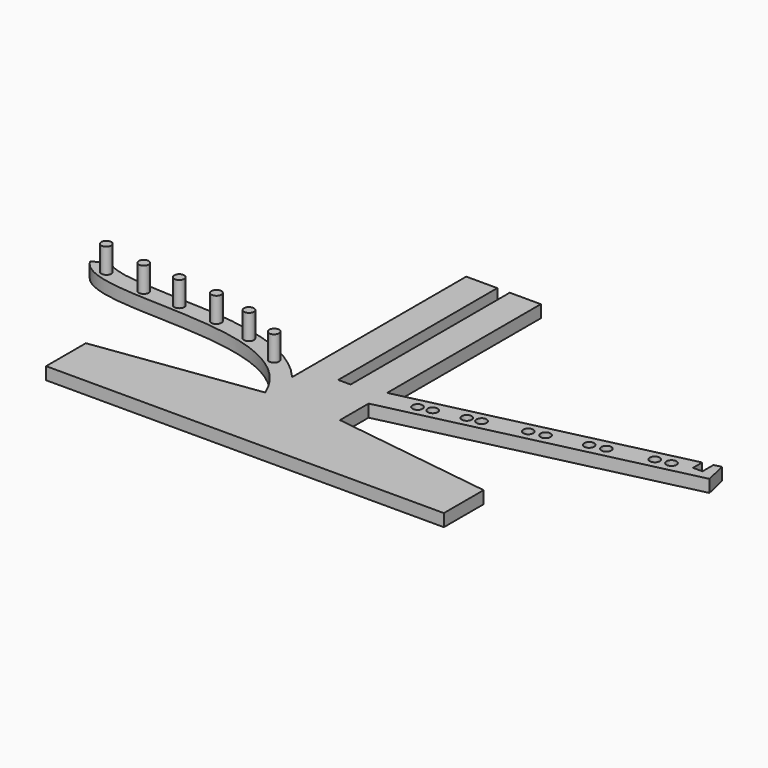
from build123d import *

# Parameters (mm, degrees)
F0_R     = 2
F1_DEPTH = 5
F2_D     = 4
F2_DEPTH = 10
F2_TIP   = 1.2017212381
F3_DEPTH = 15


# Not quite as in the source:
# - ends of sketch curves that miss each other by under 0.0002 mm in the source are joined
# - the dataset's text gives a spline's control points without its knots; the knots are read off the source's solid


with BuildPart() as f1:
    # F0 (on Top) → F1 (new body)
    with BuildSketch(Plane.XY):
        Polygon((-160, 0), (0, 0), (0, 20), (-65, 29), (-65, 43.4094795469), (-65, 52.718677739), (-65, 130), (-77.5, 130), (-77.5, 50), (-82.5, 50), (-82.5, 130), (-95, 130), (-95, 42.4402998717), (-95, 42.4395510141), (-95, 29), (-160, 20), align=None)
        with BuildLine():
            add(Edge.make_bspline(
                [(-95, 29), (-112.1026869317, 69.879398944), (-183.2138453119, 44.6590780371), (-193.7192612239, 64.3418715165)],
                knots=[0, 0, 0, 0, 104.8548540549, 104.8548540549, 104.8548540549, 104.8548540549], degree=3))
            Line((-95, 29), (-95, 42.4395510141))
            add(Edge.make_bspline(
                [(-95, 42.4395510141), (-96.2567038445, 43.9528858593), (-99.6573677898, 47.484596761), (-105.8513361132, 51.9891056969), (-113.4978559187, 55.6874902914), (-121.5446515491, 58.2622912897), (-129.8174188241, 59.9692128244), (-138.169171381, 61.0325579202), (-146.4541296432, 61.6510478997), (-154.5172718143, 62.00683513), (-162.1896252518, 62.271111182), (-169.2832883204, 62.6056387967), (-175.5824829207, 63.1564158073), (-179.9528366956, 63.8911416604), (-182.7618397147, 64.6491460265), (-184.483037472, 65.2820676907), (-185.7879555086, 65.9413674264), (-186.6785109442, 66.5698730777), (-187.2176454673, 67.115204059), (-187.4401377715, 67.4455917293), (-187.5371722477, 67.6255274527)],
                knots=[0.0840071742, 0.0840071742, 0.0840071742, 0.0840071742, 0.125, 0.1875, 0.25, 0.3125, 0.375, 0.4375, 0.5, 0.5625, 0.625, 0.6875, 0.75, 0.8125, 0.84375, 0.875, 0.90625, 0.9375, 0.96875, 0.9992998663, 0.9992998663, 0.9992998663, 0.9992998663], degree=3))
            Line((-187.5371722477, 67.6255274527), (-193.7192612239, 64.3418715165))
        make_face()
        with Locations((-185.2389183558, 61.8432959386)):
            Circle(F0_R, mode=Mode.SUBTRACT)
        with Locations((-167.974160698, 59.0616882791)):
            Circle(F0_R, mode=Mode.SUBTRACT)
        with Locations((-153.1901955605, 58.4377646446)):
            Circle(F0_R, mode=Mode.SUBTRACT)
        with Locations((-137.3645175282, 57.3560006478)):
            Circle(F0_R, mode=Mode.SUBTRACT)
        with Locations((-106.7991028057, 48.1625446324)):
            Circle(F0_R, mode=Mode.SUBTRACT)
        with Locations((-122.0965287178, 54.6330658818)):
            Circle(F0_R, mode=Mode.SUBTRACT)
        Polygon((-65, 52.718677739), (-65, 43.4094795469), (50.5995428698, 70.2936704911), (48.5456525514, 79.1252095323), (45.6876063188, 78.4605333689), (45.6876063188, 72.9172108104), (41.8661773528, 72.9172108104), (41.8661773528, 77.5718099064), align=None)
    extrude(amount=F1_DEPTH)

    # F2
    with Locations(Plane(origin=(0, 0, 0), x_dir=(1, 0, 0), z_dir=(0, 0, -1))):
        with Locations((-51.5294219104, -51.1968383797), (-46.3905660996, -52.3919467463), (-34.854432044, -55.0748261332), (-29.8337774867, -56.2424452469), (-13.9858648397, -59.9280853376), (-8.1348243559, -61.2888215973), (6.6595270344, -64.7294421898), (12.4902371317, -66.0854503512), (28.9290652415, -69.9085155886), (34.5855476759, -71.2240048204)):
            Hole(F2_D / 2, depth=F2_DEPTH)
            with Locations((0, 0, -(F2_DEPTH + F2_TIP / 2))):  # 118° drill point
                Cone(0, F2_D / 2, F2_TIP, mode=Mode.SUBTRACT)

    # F0 (on Top) → F3 (join)
    with BuildSketch(Plane.XY):
        with Locations((-106.7991028057, 48.1625446324)):
            Circle(F0_R)
        with Locations((-122.0965287178, 54.6330658818)):
            Circle(F0_R)
        with Locations((-137.3645175282, 57.3560006478)):
            Circle(F0_R)
        with Locations((-153.1901955605, 58.4377646446)):
            Circle(F0_R)
        with Locations((-167.974160698, 59.0616882791)):
            Circle(F0_R)
        with Locations((-185.2389183558, 61.8432959386)):
            Circle(F0_R)
    extrude(amount=F3_DEPTH)


solid = f1.part
